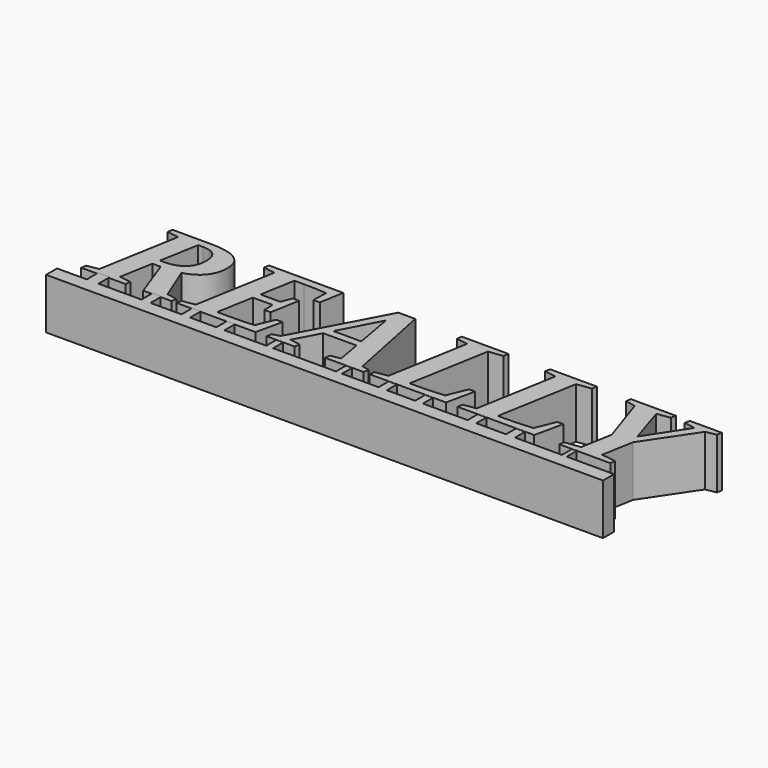
from build123d import *

# Parameters (mm, degrees)
F0_TEXT_SIZE = 28.4571058324
F1_DEPTH     = 10
F2_W         = 2.289313823
F2_H         = 2.7980539016
F2_W_2       = 1.7805807292
F2_H_2       = 2.7132639661
F2_W_3       = 0.9326860309
F2_H_3       = 2.4588960223
F2_W_4       = 1.6957912594
F2_H_4       = 2.6284744963
F2_W_5       = 1.6110017896
F2_H_5       = 2.5436845608
F2_W_6       = 1.6957893968
F2_W_7       = 1.3566315174
F2_W_8       = 1.5262113884
F2_W_9       = 1.1958102696
F2_W_10      = 1.6109999269
F3_DEPTH     = 10


# Not quite as in the source:
# - Text() gives the source's letters only with a copy of the font that has no kerning and outlines rounded to 1/6400 em; it was checked with that copy


with BuildPart() as f1:
    # F0 (on Top) → F1 (new body)
    with BuildSketch(Plane.XY):
        with Locations((-52.1448031068, 6.5565174446)):
            Text('REALLY', F0_TEXT_SIZE, font='Tinos', font_style=FontStyle.BOLDITALIC, text_align=(TextAlign.LEFT, TextAlign.BOTTOM))
    extrude(amount=F1_DEPTH)


with BuildPart() as f3:
    # F2 (on Top) → F3 (new body)
    with BuildSketch(Plane.XY):
        Polygon((-49.0843579173, 4.0467362851), (-54.9348331988, 4.0467362851), (-54.9348331988, 1.3334725518), (54.7827705741, 1.3334725518), (54.7827705741, 4.0467362851), (45.4559288919, 4.0467362851), (44.523242861, 4.0467362851), (35.281188786, 4.0467362851), (33.5006080568, 4.0467362851), (27.650134638, 4.0467362851), (25.9543452412, 4.0467362851), (17.1362366527, 4.0467362851), (15.6100252643, 4.0467362851), (10.0139193237, 4.0467362851), (8.4029193968, 4.0467362851), (1.1958102696, 4.0467362851), (0, 4.0467362851), (-12.3705081642, 4.0467362851), (-13.7271396816, 4.0467362851), (-21.9517201185, 4.0467362851), (-23.5627219081, 4.0467362851), (-28.7348795682, 4.0467362851), (-30.4306708276, 4.0467362851), (-36.535512656, 4.0467362851), (-38.3160933852, 4.0467362851), (-46.7950440943, 4.0467362851), align=None)
        with Locations((-47.9397010058, 5.4457632359)):
            Rectangle(F2_W, F2_H)
        with Locations((-37.4258030206, 5.4033682682)):
            Rectangle(F2_W_2, F2_H_2)
        with Locations((44.9895858765, 5.2761842962)):
            Rectangle(F2_W_3, F2_H_3)
        with Locations((-29.5827751979, 5.3609735332)):
            Rectangle(F2_W_4, F2_H_4)
        with Locations((34.3908984214, 5.2761842962)):
            Rectangle(F2_W_2, F2_H_3)
        with Locations((-22.7572210133, 5.3185785655)):
            Rectangle(F2_W_5, F2_H_5)
        with Locations((26.8022399396, 5.2761842962)):
            Rectangle(F2_W_6, F2_H_3)
        with Locations((-13.0488239229, 5.2761842962)):
            Rectangle(F2_W_7, F2_H_3)
        with Locations((16.3731309585, 5.2761842962)):
            Rectangle(F2_W_8, F2_H_3)
        with Locations((0.5979051348, 5.2761842962)):
            Rectangle(F2_W_9, F2_H_3)
        with Locations((9.2084193602, 5.2761842962)):
            Rectangle(F2_W_10, F2_H_3)
    extrude(amount=F3_DEPTH)


solid = Compound([f1.part, f3.part])
